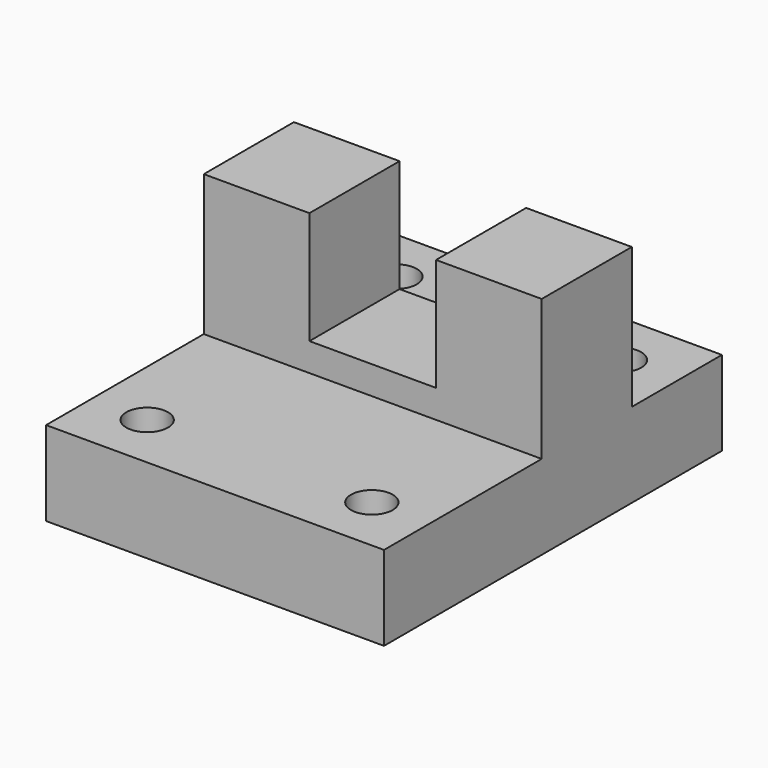
from build123d import *

# Parameters (mm, degrees)
F0_R     = 4.699
F1_DEPTH = 19.05
F2_DEPTH = 50.8
F3_DEPTH = 25.4


# Not quite as in the source:
# - a feature of the source that left no trace in its solid (it failed there, or was rolled back) is left out


with BuildPart() as f1:
    # F0 (on Top) → F1 (new body)
    with BuildSketch(Plane.XY):
        Polygon((46.0592823896, 54.4316620976), (-30.1407176104, 54.4316620976), (-30.1407176104, 29.0316620976), (-6.3155176104, 29.0316620976), (22.2340823896, 29.0316620976), (46.0592823896, 29.0316620976), align=None)
        with Locations((-17.4028014716, 41.883985333)):
            Circle(F0_R, mode=Mode.SUBTRACT)
        with Locations((33.3109036978, 41.7761531395)):
            Circle(F0_R, mode=Mode.SUBTRACT)
        Polygon((-6.3155176104, 29.0316620976), (-30.1407176104, 29.0316620976), (-30.1407176104, 3.6316620976), (-6.3155176104, 3.6316620976), (-6.3155176104, 16.6544260591), align=None)
        Polygon((-6.3155176104, 3.6316620976), (-30.1407176104, 3.6316620976), (-30.1407176104, -27.9789566994), (-30.1407176104, -40.8183379024), (-23.7907176104, -40.8183379024), (-17.4407176104, -40.8183379024), (33.3592823896, -40.8183379024), (46.0592823896, -40.8183379024), (46.0592823896, -28.1183379024), (46.0592823896, 3.6316620976), (22.2340823896, 3.6316620976), align=None)
        with Locations((-17.4763201279, -28.1499404974)):
            Circle(F0_R, mode=Mode.SUBTRACT)
        with Locations((33.0586231201, -27.9913925288)):
            Circle(F0_R, mode=Mode.SUBTRACT)
        Polygon((46.0592823896, 3.6316620976), (46.0592823896, 29.0316620976), (22.2340823896, 29.0316620976), (22.2340823896, 18.1238111109), (22.2340823896, 3.6316620976), align=None)
    extrude(amount=F1_DEPTH)

    # F0 (on Top) → F2 (join)
    with BuildSketch(Plane.XY):
        Polygon((-6.3155176104, 29.0316620976), (-30.1407176104, 29.0316620976), (-30.1407176104, 3.6316620976), (-6.3155176104, 3.6316620976), (-6.3155176104, 16.6544260591), align=None)
        Polygon((46.0592823896, 3.6316620976), (46.0592823896, 29.0316620976), (22.2340823896, 29.0316620976), (22.2340823896, 18.1238111109), (22.2340823896, 3.6316620976), align=None)
    extrude(amount=F2_DEPTH)

    # F0 (on Top) → F3 (join)
    with BuildSketch(Plane.XY):
        Polygon((22.2340823896, 29.0316620976), (-6.3155176104, 29.0316620976), (-6.3155176104, 16.6544260591), (-6.3155176104, 3.6316620976), (22.2340823896, 3.6316620976), (22.2340823896, 18.1238111109), align=None)
    extrude(amount=F3_DEPTH)


solid = f1.part
